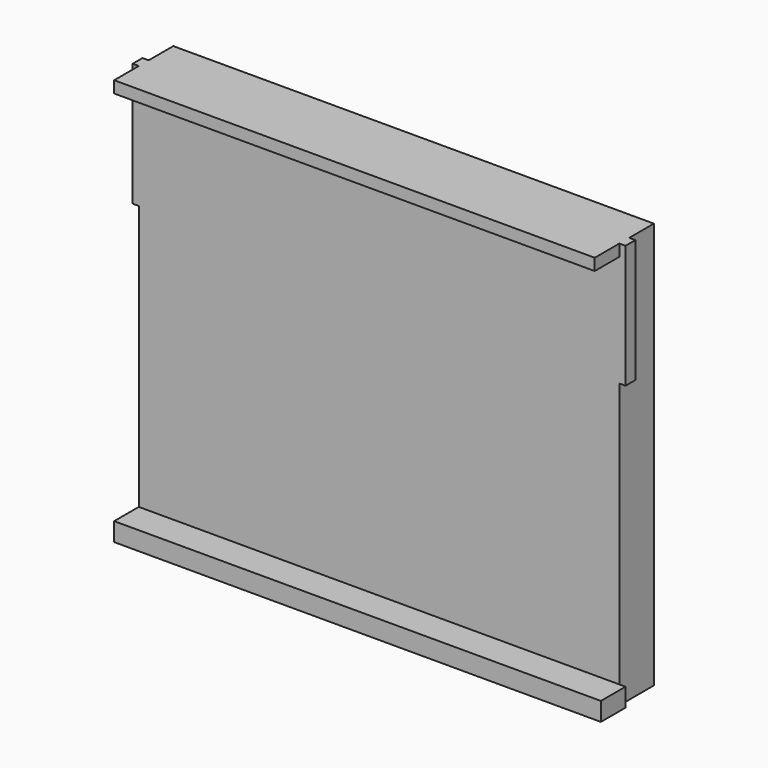
from build123d import *

# Parameters (mm, degrees)
F0_W      = 99.06
F0_H      = 80.01
F1_DEPTH  = 8.89
F3_W      = 2.54
F3_H      = 25.4
F4_DEPTH  = 1.27
F2_W      = 2.54
F2_H      = 25.4
F5_DEPTH  = 1.27
F6_W      = 85.09
F6_H      = 6.35
F7_DEPTH  = 3.81
F8_W      = 99.06
F8_H      = 2.413
F9_DEPTH  = 6.35
F10_DEPTH = 15.24


# Not quite as in the source:
# - a feature names something its author has since deleted; it is built from what else it names


with BuildPart() as f1:
    # F0 (on Front) → F1 (new body)
    with BuildSketch(Plane.XZ):
        Rectangle(F0_W, F0_H)
    extrude(amount=F1_DEPTH)

    # F3 (on face) → F4 (join)
    with BuildSketch(Plane(origin=(-49.53, 0, 0), x_dir=(0, -1, 0), z_dir=(-1, 0, 0))):
        with Locations((7.62, 27.305)):
            Rectangle(F3_W, F3_H)
    extrude(amount=F4_DEPTH)

    # F2 (on face) → F5 (join)
    with BuildSketch(Plane.YZ.offset(49.53)):
        with Locations((-7.62, 27.305)):
            Rectangle(F2_W, F2_H)
    extrude(amount=F5_DEPTH)

    # F6 (on face) → F7 (join)
    with BuildSketch(Plane(origin=(0, 0, -40.005), x_dir=(1, 0, 0), z_dir=(0, 0, -1))):
        with Locations((-6.985, 12.065)):
            Rectangle(F6_W, F6_H)
        Polygon((35.56, 8.89), (-49.53, 8.89), (-49.53, 0), (49.53, 0), (49.53, 8.89), align=None)
    extrude(amount=F7_DEPTH)

    # F8 (on face) → F9 (join)
    with BuildSketch(Plane.XZ.offset(8.89)):
        with Locations((0, 38.7985)):
            Rectangle(F8_W, F8_H)
    extrude(amount=F9_DEPTH)

    # F10 (add): a face of the model
    f10_faces = [f1.faces().sort_by_distance(p)[0] for p in [
        (35.56, -12.065, -41.91),
    ]]
    extrude(f10_faces, amount=F10_DEPTH)


solid = f1.part
